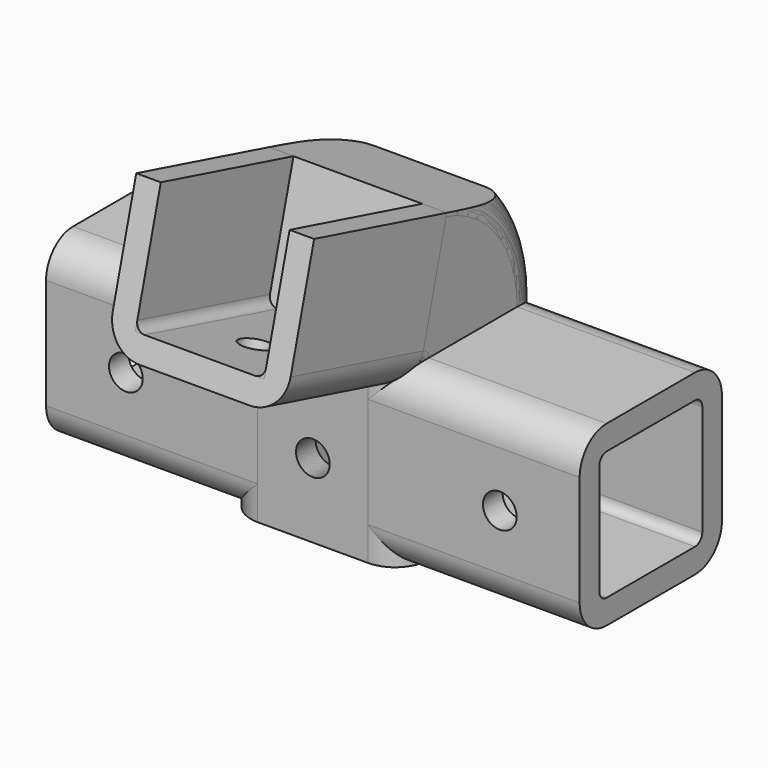
from build123d import *

# Parameters (mm, degrees)
F1_DEPTH  = 29
F3_DEPTH  = 21
F5_DEPTH  = 28
F7_DEPTH  = 28
F9_ANGLE  = 75
F11_DEPTH = 43.3
F12_R     = 2.75
F13_DEPTH = 5
F14_R     = 2.5
F15_DEPTH = 5
F16_W     = 18
F16_H     = 4
F17_DEPTH = 5.5
F18_W     = 1.5
F18_H     = 18
F19_DEPTH = 29
F21_DEPTH = 23.5
F22_R     = 2.75
F23_DEPTH = 15.2


with BuildPart() as f1:
    # F0 (on Top) → F1 (new body)
    with BuildSketch(Plane.XY):
        with BuildLine():
            Line((1.5, -4), (19.5, -4))
            ThreePointArc((19.5, -4), (23.3890872965, -2.3890872965), (25, 1.5))
            Line((25, 1.5), (25, 19.5))
            ThreePointArc((25, 19.5), (23.3890872965, 23.3890872965), (19.5, 25))
            Line((19.5, 25), (1.5, 25))
            ThreePointArc((1.5, 25), (-2.3890872965, 23.3890872965), (-4, 19.5))
            Line((-4, 19.5), (-4, 1.5))
            ThreePointArc((-4, 1.5), (-2.3890872965, -2.3890872965), (1.5, -4))
        make_face()
        with BuildLine():
            Line((19.5, 0), (1.5, 0))
            ThreePointArc((1.5, 0), (0.4393398282, 0.4393398282), (0, 1.5))
            Line((0, 1.5), (0, 19.5))
            ThreePointArc((0, 19.5), (0.4393398282, 20.5606601718), (1.5, 21))
            Line((1.5, 21), (19.5, 21))
            ThreePointArc((19.5, 21), (20.5606601718, 20.5606601718), (21, 19.5))
            Line((21, 19.5), (21, 1.5))
            ThreePointArc((21, 1.5), (20.5606601718, 0.4393398282), (19.5, 0))
        make_face(mode=Mode.SUBTRACT)
    extrude(amount=-F1_DEPTH)

    # F12 (on face) → F13 (cut)
    with BuildSketch(Plane.XZ.offset(4)):
        with Locations((10.5, -16.8672984689)):
            Circle(F12_R)
    extrude(amount=-F13_DEPTH, mode=Mode.SUBTRACT)


with BuildPart() as f3:
    # F2 (on Right) → F3 (new body)
    with BuildSketch(Plane.YZ):
        Polygon((-27.0459231361, 7.2469332629), (0, 0), (5.1763809021, 19.3185165258), (-21.869542234, 26.5654497887), align=None)
    extrude(amount=F3_DEPTH)

    # F6 (on face) → F7 (cut)
    with BuildSketch(Plane(origin=(0, -27.0459231361, 7.2469332629), x_dir=(1, 0, 0), z_dir=(0, -0.9659258263, 0.2588190451))):
        with BuildLine():
            Line((21, 20), (0, 20))
            Line((0, 20), (0, 1.5))
            ThreePointArc((0, 1.5), (0.4393398282, 0.4393398282), (1.5, 0))
            Line((1.5, 0), (19.5, 0))
            ThreePointArc((19.5, 0), (20.5606601718, 0.4393398282), (21, 1.5))
            Line((21, 1.5), (21, 20))
        make_face()
    extrude(amount=-F7_DEPTH, mode=Mode.SUBTRACT)


with BuildPart() as f5:
    # F4 (on face) → F5 (new body)
    with BuildSketch(Plane(origin=(0, -27.0459231361, 7.2469332629), x_dir=(1, 0, 0), z_dir=(0, -0.9659258263, 0.2588190451))):
        with BuildLine():
            Line((0, 1.5), (0, 20))
            Line((0, 20), (-4, 20))
            Line((-4, 20), (-4, 1.5))
            ThreePointArc((-4, 1.5), (-2.3890872965, -2.3890872965), (1.5, -4))
            Line((1.5, -4), (19.5, -4))
            ThreePointArc((19.5, -4), (23.3890872965, -2.3890872965), (25, 1.5))
            Line((25, 1.5), (25, 20))
            Line((25, 20), (21, 20))
            Line((21, 20), (21, 1.5))
            Line((21, 1.5), (21, 0))
            Line((21, 0), (19.5, 0))
            Line((19.5, 0), (1.5, 0))
            Line((1.5, 0), (0, 0))
            Line((0, 0), (0, 1.5))
        make_face()
    extrude(amount=-F5_DEPTH)

    # F14 (on face) → F15 (cut)
    with BuildSketch(Plane(origin=(0, -1.0352761804, -3.8637033052), x_dir=(1, 0, 0), z_dir=(0, -0.2588190451, -0.9659258263))):
        with Locations((10.5, 16.148366034)):
            Circle(F14_R)
    extrude(amount=-F15_DEPTH, mode=Mode.SUBTRACT)


with BuildPart() as f9:
    # F8 (on face) → F9 (revolve)
    with BuildSketch(Plane.XY):
        with BuildLine():
            ThreePointArc((0, 19.5), (0.4393398282, 20.5606601718), (1.5, 21))
            Line((1.5, 21), (19.5, 21))
            ThreePointArc((19.5, 21), (20.5606601718, 20.5606601718), (21, 19.5))
            Line((21, 19.5), (21, 1.5))
            ThreePointArc((21, 1.5), (20.5606601718, 0.4393398282), (19.5, 0))
            Line((19.5, 0), (24.7915026221, 0))
            ThreePointArc((24.7915026221, 0), (24.9476262914, 0.7427894684), (25, 1.5))
            Line((25, 1.5), (25, 19.5))
            ThreePointArc((25, 19.5), (23.3890872965, 23.3890872965), (19.5, 25))
            Line((19.5, 25), (1.5, 25))
            ThreePointArc((1.5, 25), (-2.3890872965, 23.3890872965), (-4, 19.5))
            Line((-4, 19.5), (-4, 1.5))
            ThreePointArc((-4, 1.5), (-3.9476262914, 0.7427894684), (-3.7915026221, 0))
            Line((-3.7915026221, 0), (1.5, 0))
            ThreePointArc((1.5, 0), (0.4393398282, 0.4393398282), (0, 1.5))
            Line((0, 1.5), (0, 19.5))
        make_face()
        with BuildLine():
            Line((19.5, 21), (1.5, 21))
            ThreePointArc((1.5, 21), (0.4393398282, 20.5606601718), (0, 19.5))
            Line((0, 19.5), (0, 1.5))
            ThreePointArc((0, 1.5), (0.4393398282, 0.4393398282), (1.5, 0))
            Line((1.5, 0), (19.5, 0))
            ThreePointArc((19.5, 0), (20.5606601718, 0.4393398282), (21, 1.5))
            Line((21, 1.5), (21, 19.5))
            ThreePointArc((21, 19.5), (20.5606601718, 20.5606601718), (19.5, 21))
        make_face()
    revolve(axis=Axis((10.5, 0, 0), (1, 0, 0)), revolution_arc=F9_ANGLE)

    # F10 (on face) → F11 (cut)
    with BuildSketch(Plane(origin=(-4, 0, 0), x_dir=(0, -1, 0), z_dir=(-1, 0, 0))):
        Polygon((-21.5909180111, 14.9202545633), (-5.1763809021, 19.3185165258), (-5.1763809021, 24.5526935905), (-23.506142199, 23.2962071896), align=None)
    extrude(amount=-F11_DEPTH, mode=Mode.SUBTRACT)


with BuildPart() as f17:
    # F16 (on face) → F17 (new body, symmetric)
    with BuildSketch(Plane.YZ.offset(25)):
        with Locations((10.5, -2)):
            Rectangle(F16_W, F16_H)
        with Locations((10.5, -27)):
            Rectangle(F16_W, F16_H)
        with BuildLine():
            ThreePointArc((-4, -23.5), (-2.3890872965, -27.3890872965), (1.5, -29))
            Line((1.5, -29), (1.5, -25))
            ThreePointArc((1.5, -25), (0.4393398282, -24.5606601718), (0, -23.5))
            Line((0, -23.5), (0, -5.5))
            ThreePointArc((0, -5.5), (0.4393398282, -4.4393398282), (1.5, -4))
            Line((1.5, -4), (1.5, 0))
            ThreePointArc((1.5, 0), (-2.3890872965, -1.6109127035), (-4, -5.5))
            Line((-4, -5.5), (-4, -23.5))
        make_face()
        with BuildLine():
            Line((19.5, -25), (19.5, -29))
            ThreePointArc((19.5, -29), (23.3890872965, -27.3890872965), (25, -23.5))
            Line((25, -23.5), (25, -5.5))
            ThreePointArc((25, -5.5), (23.3890872965, -1.6109127035), (19.5, 0))
            Line((19.5, 0), (19.5, -4))
            ThreePointArc((19.5, -4), (20.5606601718, -4.4393398282), (21, -5.5))
            Line((21, -5.5), (21, -23.5))
            ThreePointArc((21, -23.5), (20.5606601718, -24.5606601718), (19.5, -25))
        make_face()
    extrude(amount=F17_DEPTH, both=True)

    # F18 (on face) → F19 (cut)
    with BuildSketch(Plane(origin=(0, 0, -29), x_dir=(1, 0, 0), z_dir=(0, 0, -1))):
        with BuildLine():
            ThreePointArc((21, -1.5), (20.5606601718, -0.4393398282), (19.5, 0))
            Line((19.5, 0), (19.5, -1.5))
            Line((19.5, -1.5), (21, -1.5))
        make_face()
        with Locations((20.25, -10.5)):
            Rectangle(F18_W, F18_H)
        with BuildLine():
            Line((21, -19.5), (19.5, -19.5))
            Line((19.5, -19.5), (19.5, -21))
            ThreePointArc((19.5, -21), (20.5606601718, -20.5606601718), (21, -19.5))
        make_face()
    extrude(amount=-F19_DEPTH, mode=Mode.SUBTRACT)

    # F20 (on face) → F21 (join)
    with BuildSketch(Plane.YZ.offset(30.5)):
        with BuildLine():
            Line((25, -23.5), (25, -5.5))
            ThreePointArc((25, -5.5), (23.3890872965, -1.6109127035), (19.5, 0))
            Line((19.5, 0), (1.5, 0))
            ThreePointArc((1.5, 0), (-2.3890872965, -1.6109127035), (-4, -5.5))
            Line((-4, -5.5), (-4, -23.5))
            ThreePointArc((-4, -23.5), (-2.3890872965, -27.3890872965), (1.5, -29))
            Line((1.5, -29), (19.5, -29))
            ThreePointArc((19.5, -29), (23.3890872965, -27.3890872965), (25, -23.5))
        make_face()
        with BuildLine():
            Line((19.5, -25), (1.5, -25))
            ThreePointArc((1.5, -25), (0.4393398282, -24.5606601718), (0, -23.5))
            Line((0, -23.5), (0, -5.5))
            ThreePointArc((0, -5.5), (0.4393398282, -4.4393398282), (1.5, -4))
            Line((1.5, -4), (19.5, -4))
            ThreePointArc((19.5, -4), (20.5606601718, -4.4393398282), (21, -5.5))
            Line((21, -5.5), (21, -23.5))
            ThreePointArc((21, -23.5), (20.5606601718, -24.5606601718), (19.5, -25))
        make_face(mode=Mode.SUBTRACT)
    extrude(amount=F21_DEPTH)

    # F22 (on face) → F23 (cut)
    with BuildSketch(Plane.XZ.offset(4)):
        with Locations((40.9836284816, -14.5)):
            Circle(F22_R)
    extrude(amount=-F23_DEPTH, mode=Mode.SUBTRACT)


with BuildPart() as f25_1:
    # F25: instance of F17
    add(f17.part.mirror(Plane.YZ.offset(10.5)))


with BuildPart() as f25_2:
    # F25: instance of F1
    add(f1.part.mirror(Plane.YZ.offset(10.5)))


with BuildPart() as f25_3:
    # F25: instance of F9
    add(f9.part.mirror(Plane.YZ.offset(10.5)))


solid = Compound([f1.part, f3.part, f5.part, f9.part, f17.part, f25_1.part, f25_2.part, f25_3.part])
